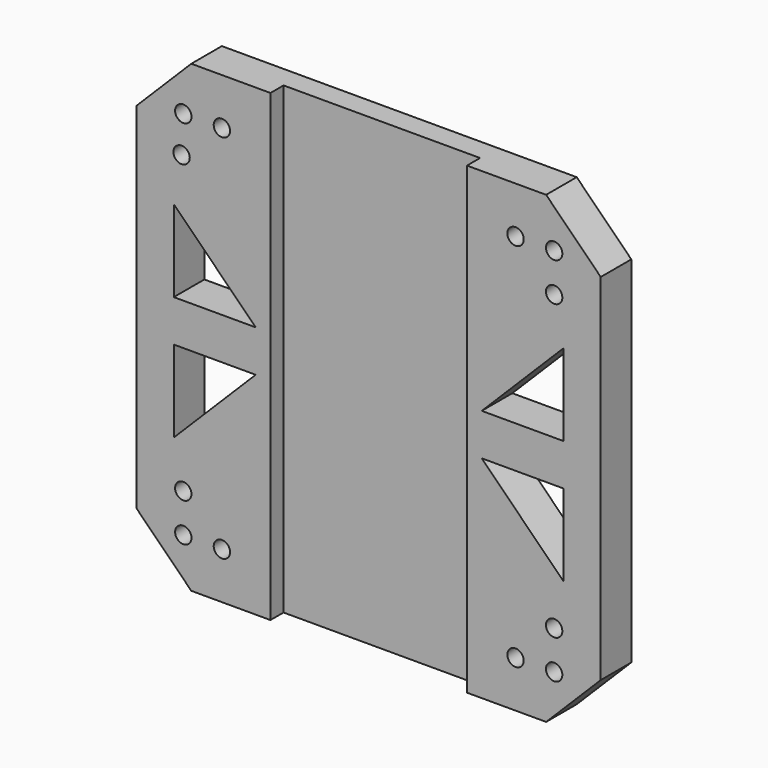
from build123d import *

# Parameters (mm, degrees)
F0_R     = 1.5
F0_W     = 36
F0_H     = 85
F1_DEPTH = 4
F2_SIZE  = 10
F3_DEPTH = 7


with BuildPart() as f1:
    # F0 (on Front) → F1 (new body)
    with BuildSketch(Plane.XZ):
        Polygon((42.5, 32.5), (42.5, 42.5), (37.5, 37.5), align=None)
        Polygon((37.5, 37.5), (42.5, 42.5), (32.5, 42.5), align=None)
        Polygon((42.5, -32.5), (42.5, 32.5), (37.5, 37.5), (32.5, 42.5), (18, 42.5), (18, -42.5), (32.5, -42.5), (37.5, -37.5), align=None)
        with Locations((26.8933982822, -33.9644660941)):
            Circle(F0_R, mode=Mode.SUBTRACT)
        with BuildLine():
            ThreePointArc((35.4644660941, -33.9644660941), (35.3502853928, -34.5384912426), (35.0251262658, -35.0251262658))
            ThreePointArc((35.0251262658, -35.0251262658), (32.9038059223, -35.0251262658), (32.9038059223, -32.9038059223))
            ThreePointArc((32.9038059223, -32.9038059223), (34.5384912426, -32.5786467953), (35.4644660941, -33.9644660941))
        make_face(mode=Mode.SUBTRACT)
        with Locations((33.9644660941, -26.8933982822)):
            Circle(F0_R, mode=Mode.SUBTRACT)
        Polygon((20.7055291533, -3.823871389), (35.7055291533, -3.823871389), (35.7055291533, -18.823871389), align=None, mode=Mode.SUBTRACT)
        Polygon((35.7055291533, 3.823871389), (20.7055291533, 3.823871389), (35.7055291533, 18.823871389), align=None, mode=Mode.SUBTRACT)
        with BuildLine():
            ThreePointArc((35.4644660941, 26.8933982822), (33.3904409455, 25.5075789834), (32.9038059223, 27.954058454))
            ThreePointArc((32.9038059223, 27.954058454), (34.5384912426, 28.279217581), (35.4644660941, 26.8933982822))
        make_face(mode=Mode.SUBTRACT)
        with BuildLine():
            ThreePointArc((28.3933982822, 33.9644660941), (28.279217581, 33.3904409455), (27.954058454, 32.9038059223))
            ThreePointArc((27.954058454, 32.9038059223), (25.5075789834, 34.5384912426), (28.3933982822, 33.9644660941))
        make_face(mode=Mode.SUBTRACT)
        with BuildLine():
            ThreePointArc((32.9038059223, 32.9038059223), (32.9038059223, 35.0251262658), (35.0251262658, 35.0251262658))
            ThreePointArc((35.0251262658, 35.0251262658), (35.3502853928, 34.5384912426), (35.4644660941, 33.9644660941))
            ThreePointArc((35.4644660941, 33.9644660941), (34.5384912426, 32.5786467953), (32.9038059223, 32.9038059223))
        make_face(mode=Mode.SUBTRACT)
        Polygon((42.5, -42.5), (42.5, -32.5), (37.5, -37.5), align=None)
        Rectangle(F0_W, F0_H)
        Polygon((32.5, -42.5), (42.5, -42.5), (37.5, -37.5), align=None)
        Polygon((-18, -42.5), (-18, 42.5), (-32.5, 42.5), (-37.5, 37.5), (-42.5, 32.5), (-42.5, -32.5), (-37.5, -37.5), (-32.5, -42.5), align=None)
        with BuildLine():
            ThreePointArc((-32.4644660941, -33.9644660941), (-33.3904409455, -35.3502853928), (-35.0251262658, -35.0251262658))
            ThreePointArc((-35.0251262658, -35.0251262658), (-35.0251262658, -32.9038059223), (-32.9038059223, -32.9038059223))
            ThreePointArc((-32.9038059223, -32.9038059223), (-32.5786467953, -33.3904409455), (-32.4644660941, -33.9644660941))
        make_face(mode=Mode.SUBTRACT)
        with Locations((-26.8933982822, -33.9644660941)):
            Circle(F0_R, mode=Mode.SUBTRACT)
        with Locations((-33.9644660941, -26.8933982822)):
            Circle(F0_R, mode=Mode.SUBTRACT)
        Polygon((-20.7055291533, -3.823871389), (-35.7055291533, -18.823871389), (-35.7055291533, -3.823871389), align=None, mode=Mode.SUBTRACT)
        Polygon((-35.7055291533, 3.823871389), (-35.7055291533, 18.823871389), (-20.7055291533, 3.823871389), align=None, mode=Mode.SUBTRACT)
        with BuildLine():
            ThreePointArc((-32.7795228992, 27.2231633162), (-35.6780717969, 26.6808894181), (-33.1716042066, 28.2343587329))
            ThreePointArc((-33.1716042066, 28.2343587329), (-32.8809740014, 27.7654372144), (-32.7795228992, 27.2231633162))
        make_face(mode=Mode.SUBTRACT)
        with BuildLine():
            ThreePointArc((-32.9038059223, 32.9038059223), (-35.0251262658, 32.9038059223), (-35.0251262658, 35.0251262658))
            ThreePointArc((-35.0251262658, 35.0251262658), (-33.3904409455, 35.3502853928), (-32.4644660941, 33.9644660941))
            ThreePointArc((-32.4644660941, 33.9644660941), (-32.5786467953, 33.3904409455), (-32.9038059223, 32.9038059223))
        make_face(mode=Mode.SUBTRACT)
        with BuildLine():
            ThreePointArc((-25.3933982822, 33.9644660941), (-26.3511243841, 32.5659171963), (-28.0013169747, 32.9532706774))
            ThreePointArc((-28.0013169747, 32.9532706774), (-27.4356721803, 35.3630149918), (-25.3933982822, 33.9644660941))
        make_face(mode=Mode.SUBTRACT)
        Polygon((-37.5, 37.5), (-32.5, 42.5), (-42.5, 42.5), align=None)
        Polygon((-42.5, 32.5), (-37.5, 37.5), (-42.5, 42.5), align=None)
        Polygon((-42.5, -42.5), (-32.5, -42.5), (-37.5, -37.5), align=None)
        Polygon((-42.5, -42.5), (-37.5, -37.5), (-42.5, -32.5), align=None)
    extrude(amount=F1_DEPTH)

    # F2
    f2_edges = [f1.edges().sort_by_distance(p)[0] for p in [
        (42.5, -2, 42.5),
        (-42.5, -2, 42.5),
        (-42.5, -2, -42.5),
        (42.5, -2, -42.5),
    ]]
    chamfer(f2_edges, length=F2_SIZE)

    # F0 (on Front) → F3 (join)
    with BuildSketch(Plane.XZ):
        Polygon((-18, -42.5), (-18, 42.5), (-32.5, 42.5), (-37.5, 37.5), (-42.5, 32.5), (-42.5, -32.5), (-37.5, -37.5), (-32.5, -42.5), align=None)
        with BuildLine():
            ThreePointArc((-32.4644660941, -33.9644660941), (-33.3904409455, -35.3502853928), (-35.0251262658, -35.0251262658))
            ThreePointArc((-35.0251262658, -35.0251262658), (-35.0251262658, -32.9038059223), (-32.9038059223, -32.9038059223))
            ThreePointArc((-32.9038059223, -32.9038059223), (-32.5786467953, -33.3904409455), (-32.4644660941, -33.9644660941))
        make_face(mode=Mode.SUBTRACT)
        with Locations((-26.8933982822, -33.9644660941)):
            Circle(F0_R, mode=Mode.SUBTRACT)
        with Locations((-33.9644660941, -26.8933982822)):
            Circle(F0_R, mode=Mode.SUBTRACT)
        Polygon((-20.7055291533, -3.823871389), (-35.7055291533, -18.823871389), (-35.7055291533, -3.823871389), align=None, mode=Mode.SUBTRACT)
        Polygon((-35.7055291533, 3.823871389), (-35.7055291533, 18.823871389), (-20.7055291533, 3.823871389), align=None, mode=Mode.SUBTRACT)
        with BuildLine():
            ThreePointArc((-32.7795228992, 27.2231633162), (-35.6780717969, 26.6808894181), (-33.1716042066, 28.2343587329))
            ThreePointArc((-33.1716042066, 28.2343587329), (-32.8809740014, 27.7654372144), (-32.7795228992, 27.2231633162))
        make_face(mode=Mode.SUBTRACT)
        with BuildLine():
            ThreePointArc((-32.9038059223, 32.9038059223), (-35.0251262658, 32.9038059223), (-35.0251262658, 35.0251262658))
            ThreePointArc((-35.0251262658, 35.0251262658), (-33.3904409455, 35.3502853928), (-32.4644660941, 33.9644660941))
            ThreePointArc((-32.4644660941, 33.9644660941), (-32.5786467953, 33.3904409455), (-32.9038059223, 32.9038059223))
        make_face(mode=Mode.SUBTRACT)
        with BuildLine():
            ThreePointArc((-25.3933982822, 33.9644660941), (-26.3511243841, 32.5659171963), (-28.0013169747, 32.9532706774))
            ThreePointArc((-28.0013169747, 32.9532706774), (-27.4356721803, 35.3630149918), (-25.3933982822, 33.9644660941))
        make_face(mode=Mode.SUBTRACT)
        Polygon((42.5, -32.5), (42.5, 32.5), (37.5, 37.5), (32.5, 42.5), (18, 42.5), (18, -42.5), (32.5, -42.5), (37.5, -37.5), align=None)
        with Locations((26.8933982822, -33.9644660941)):
            Circle(F0_R, mode=Mode.SUBTRACT)
        with BuildLine():
            ThreePointArc((35.4644660941, -33.9644660941), (35.3502853928, -34.5384912426), (35.0251262658, -35.0251262658))
            ThreePointArc((35.0251262658, -35.0251262658), (32.9038059223, -35.0251262658), (32.9038059223, -32.9038059223))
            ThreePointArc((32.9038059223, -32.9038059223), (34.5384912426, -32.5786467953), (35.4644660941, -33.9644660941))
        make_face(mode=Mode.SUBTRACT)
        with Locations((33.9644660941, -26.8933982822)):
            Circle(F0_R, mode=Mode.SUBTRACT)
        Polygon((20.7055291533, -3.823871389), (35.7055291533, -3.823871389), (35.7055291533, -18.823871389), align=None, mode=Mode.SUBTRACT)
        Polygon((35.7055291533, 3.823871389), (20.7055291533, 3.823871389), (35.7055291533, 18.823871389), align=None, mode=Mode.SUBTRACT)
        with BuildLine():
            ThreePointArc((35.4644660941, 26.8933982822), (33.3904409455, 25.5075789834), (32.9038059223, 27.954058454))
            ThreePointArc((32.9038059223, 27.954058454), (34.5384912426, 28.279217581), (35.4644660941, 26.8933982822))
        make_face(mode=Mode.SUBTRACT)
        with BuildLine():
            ThreePointArc((28.3933982822, 33.9644660941), (28.279217581, 33.3904409455), (27.954058454, 32.9038059223))
            ThreePointArc((27.954058454, 32.9038059223), (25.5075789834, 34.5384912426), (28.3933982822, 33.9644660941))
        make_face(mode=Mode.SUBTRACT)
        with BuildLine():
            ThreePointArc((32.9038059223, 32.9038059223), (32.9038059223, 35.0251262658), (35.0251262658, 35.0251262658))
            ThreePointArc((35.0251262658, 35.0251262658), (35.3502853928, 34.5384912426), (35.4644660941, 33.9644660941))
            ThreePointArc((35.4644660941, 33.9644660941), (34.5384912426, 32.5786467953), (32.9038059223, 32.9038059223))
        make_face(mode=Mode.SUBTRACT)
    extrude(amount=F3_DEPTH)


solid = f1.part
